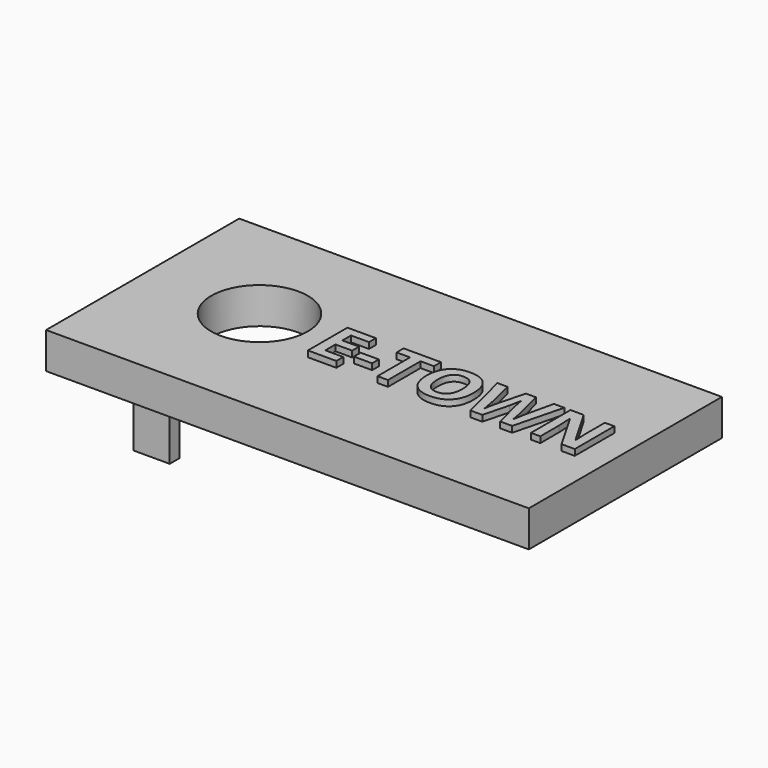
from build123d import *

# Parameters (mm, degrees)
F0_W         = 101.6
F0_H         = 50.8
F0_R         = 10.16
F1_DEPTH     = 7.62
F2_T         = -2.54
F3_W         = 7.62
F3_H         = 15.24
F3_R         = 1.397
F4_DEPTH     = 2.54
F5_TEXT_SIZE = 14.5629041053
F6_DEPTH     = 1.27


# Not quite as in the source:
# - Text() gives the source's letters only with a copy of the font that has no kerning and outlines rounded to 1/6400 em; it was checked with that copy


with BuildPart() as f1:
    # F0 (on Top) → F1 (new body)
    with BuildSketch(Plane.XY):
        with Locations((4.6097417189, 6.1076339334)):
            Rectangle(F0_W, F0_H)
        with Locations((-22.4455539137, 7.1764695458)):
            Circle(F0_R, mode=Mode.SUBTRACT)
    extrude(amount=F1_DEPTH)

    # F2
    f2_openings = [f1.faces().sort_by_distance(p)[0] for p in [
        (6.423647, 6.035975, 0),
    ]]
    offset(amount=F2_T, openings=f2_openings)

    # F5 (on face) → F6 (join)
    with BuildSketch(Plane.XY.offset(7.62)):
        with Locations((-7.8292112215, 0)):
            Text('E-TOWN', F5_TEXT_SIZE, font='Open Sans', font_style=FontStyle.BOLD, text_align=(TextAlign.LEFT, TextAlign.BOTTOM))
    extrude(amount=F6_DEPTH)


with BuildPart() as f4:
    # F3 (on Front) → F4 (new body)
    with BuildSketch(Plane.XZ):
        with Locations((-37.3850930482, -12.2705919779)):
            Rectangle(F3_W, F3_H)
        with Locations((-37.6225449145, -7.1926321834)):
            Circle(F3_R, mode=Mode.SUBTRACT)
    extrude(amount=F4_DEPTH)


solid = Compound([f1.part, f4.part])
